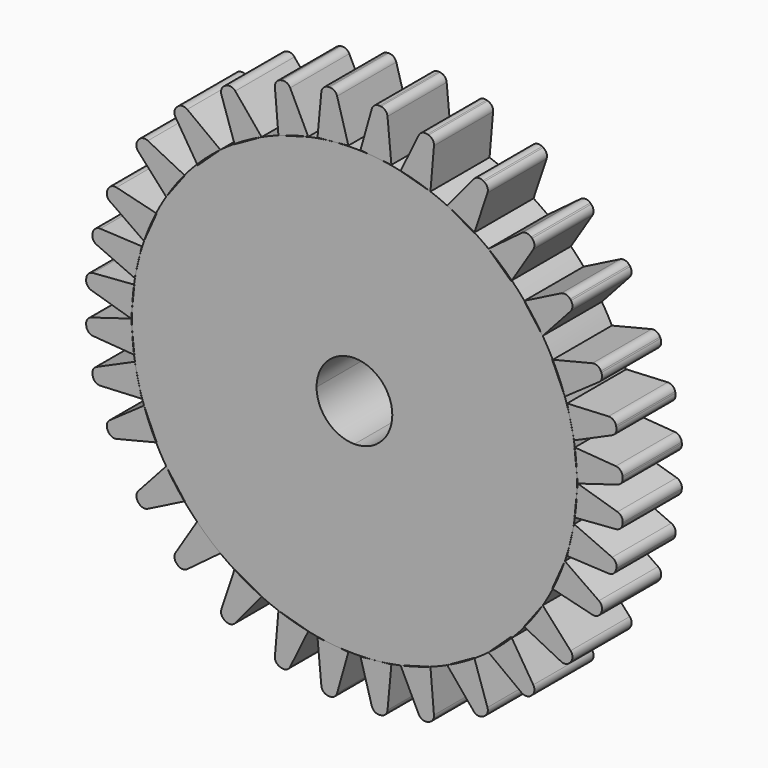
from build123d import *

# Parameters (mm, degrees)
F1_DEPTH = 12.7
F2_DEPTH = 12.7


# Not quite as in the source:
# - a feature names something its author has since deleted; it is built from what else it names


with BuildPart() as f1:
    # F0 (on Front) → F1 (new body)
    with BuildSketch(Plane.XZ):
        with BuildLine():
            Line((6.5054095145, 0), (38.2263594969, 0))
            ThreePointArc((38.2263594969, 0), (38.2190910967, 0.7454100379), (38.1972886603, 1.4905366096))
            Line((38.1972886603, 1.4905366096), (37.8051740161, 5.3060541003))
            Line((37.8051740161, 5.3060541003), (37.8568663972, 5.3020964693))
            ThreePointArc((37.8568663972, 5.3020964693), (37.7123171402, 6.247855336), (37.5441442564, 7.1897004415))
            Line((37.5441442564, 7.1897004415), (36.8769989926, 10.0668518258))
            ThreePointArc((36.8769989926, 10.0668518258), (36.5302837796, 11.2602365592), (36.1449602441, 12.4417205133))
            Line((36.1449602441, 12.4417205133), (33.966945199, 17.3107867958))
            Line((33.966945199, 17.3107867958), (34.0692924567, 17.3360281461))
            ThreePointArc((34.0692924567, 17.3360281461), (33.2407623999, 18.8760768026), (32.3426638377, 20.3766203347))
            Line((32.3426638377, 20.3766203347), (29.136457273, 24.6303906457))
            Line((29.136457273, 24.6303906457), (29.2045556993, 24.6647215023))
            ThreePointArc((29.2045556993, 24.6647215023), (28.1414113561, 25.8711330882), (27.0284704993, 27.0317654409))
            Line((27.0284704993, 27.0317654409), (26.9292951534, 26.873760444))
            Line((26.9292951534, 26.873760444), (23.028254509, 30.5115396965))
            ThreePointArc((23.028254509, 30.5115396965), (21.8357551707, 31.3760156251), (20.6108385483, 32.193910833))
            Line((20.6108385483, 32.193910833), (20.5898791317, 32.1310935588))
            Line((20.5898791317, 32.1310935588), (15.9399155527, 34.7444046223))
            ThreePointArc((15.9399155527, 34.7444046223), (14.4762769158, 35.3792589951), (12.9874228564, 35.9524882022))
            Line((12.9874228564, 35.9524882022), (7.9227071255, 37.3802185059))
            Line((7.9227071255, 37.3802185059), (7.9298244174, 37.3948184257))
            ThreePointArc((7.9298244174, 37.3948184257), (6.2217980358, 37.7166248435), (4.5009090674, 37.960458084))
            Line((4.5009090674, 37.960458084), (2.9038043086, 38.1159085018))
            ThreePointArc((2.9038043086, 38.1159085018), (0, 38.2263594969), (-2.9038043086, 38.1159085018))
            Line((-2.9038043086, 38.1159085018), (-4.5009090674, 37.960458084))
            ThreePointArc((-4.5009090674, 37.960458084), (-6.2217980358, 37.7166248435), (-7.9298244174, 37.3948184257))
            Line((-7.9298244174, 37.3948184257), (-7.9227071255, 37.3802185059))
            Line((-7.9227071255, 37.3802185059), (-12.9874228564, 35.9524882022))
            ThreePointArc((-12.9874228564, 35.9524882022), (-14.4762769158, 35.3792589951), (-15.9399155527, 34.7444046223))
            Line((-15.9399155527, 34.7444046223), (-20.5898791317, 32.1310935588))
            Line((-20.5898791317, 32.1310935588), (-20.6108385483, 32.193910833))
            ThreePointArc((-20.6108385483, 32.193910833), (-21.8357551707, 31.3760156251), (-23.028254509, 30.5115396965))
            Line((-23.028254509, 30.5115396965), (-26.9292951534, 26.873760444))
            Line((-26.9292951534, 26.873760444), (-27.0284704993, 27.0317654409))
            ThreePointArc((-27.0284704993, 27.0317654409), (-28.1414113561, 25.8711330882), (-29.2045556993, 24.6647215023))
            Line((-29.2045556993, 24.6647215023), (-29.136457273, 24.6303906457))
            Line((-29.136457273, 24.6303906457), (-32.3426638377, 20.3766203347))
            ThreePointArc((-32.3426638377, 20.3766203347), (-33.2407623999, 18.8760768026), (-34.0692924567, 17.3360281461))
            Line((-34.0692924567, 17.3360281461), (-33.966945199, 17.3107867958))
            Line((-33.966945199, 17.3107867958), (-36.1449602441, 12.4417205133))
            ThreePointArc((-36.1449602441, 12.4417205133), (-36.5302837796, 11.2602365592), (-36.8769989926, 10.0668518258))
            Line((-36.8769989926, 10.0668518258), (-37.5441442564, 7.1897004415))
            ThreePointArc((-37.5441442564, 7.1897004415), (-37.7123171402, 6.247855336), (-37.8568663972, 5.3020964693))
            Line((-37.8568663972, 5.3020964693), (-37.8051740161, 5.3060541003))
            Line((-37.8051740161, 5.3060541003), (-38.1972886603, 1.4905366096))
            ThreePointArc((-38.1972886603, 1.4905366096), (-38.2190910967, 0.7454100379), (-38.2263594969, 0))
            Line((-38.2263594969, 0), (-6.5054095145, 0))
            ThreePointArc((-6.5054095145, 0), (-4.6000191821, 4.6000191821), (0, 6.5054095145))
            ThreePointArc((0, 6.5054095145), (4.6000191821, 4.6000191821), (6.5054095145, 0))
        make_face()
        with BuildLine():
            Line((0, -38.2263594969), (0, -6.5054095145))
            ThreePointArc((0, -6.5054095145), (-4.6000191821, -4.6000191821), (-6.5054095145, 0))
            Line((-6.5054095145, 0), (-38.2263594969, 0))
            ThreePointArc((-38.2263594969, 0), (-38.2190910967, -0.7454100379), (-38.1972886603, -1.4905366096))
            Line((-38.1972886603, -1.4905366096), (-37.8051740161, -5.3060541003))
            Line((-37.8051740161, -5.3060541003), (-37.8568663972, -5.3020964693))
            ThreePointArc((-37.8568663972, -5.3020964693), (-37.7123171402, -6.247855336), (-37.5441442564, -7.1897004415))
            Line((-37.5441442564, -7.1897004415), (-36.8769989926, -10.0668518258))
            ThreePointArc((-36.8769989926, -10.0668518258), (-36.5302837796, -11.2602365592), (-36.1449602441, -12.4417205133))
            Line((-36.1449602441, -12.4417205133), (-33.966945199, -17.3107867958))
            Line((-33.966945199, -17.3107867958), (-34.0692924567, -17.3360281461))
            ThreePointArc((-34.0692924567, -17.3360281461), (-33.2407623999, -18.8760768026), (-32.3426638377, -20.3766203347))
            Line((-32.3426638377, -20.3766203347), (-29.136457273, -24.6303906457))
            Line((-29.136457273, -24.6303906457), (-29.2045556993, -24.6647215023))
            ThreePointArc((-29.2045556993, -24.6647215023), (-28.1414113561, -25.8711330882), (-27.0284704993, -27.0317654409))
            ThreePointArc((-27.0284704993, -27.0317654409), (-25.0887651521, -28.8410891529), (-23.028254509, -30.5115396965))
            ThreePointArc((-23.028254509, -30.5115396965), (-21.8357551707, -31.3760156251), (-20.6108385483, -32.193910833))
            Line((-20.6108385483, -32.193910833), (-20.5898791317, -32.1310935588))
            Line((-20.5898791317, -32.1310935588), (-15.9399155527, -34.7444046223))
            ThreePointArc((-15.9399155527, -34.7444046223), (-14.4762769158, -35.3792589951), (-12.9874228564, -35.9524882022))
            Line((-12.9874228564, -35.9524882022), (-7.9227071255, -37.3802185059))
            Line((-7.9227071255, -37.3802185059), (-7.9298244174, -37.3948184257))
            ThreePointArc((-7.9298244174, -37.3948184257), (-6.2217980358, -37.7166248435), (-4.5009090674, -37.960458084))
            Line((-4.5009090674, -37.960458084), (-2.9038043086, -38.1159085018))
            ThreePointArc((-2.9038043086, -38.1159085018), (-1.4529520712, -38.1987367679), (0, -38.2263594969))
        make_face()
        with BuildLine():
            ThreePointArc((38.1972886603, -1.4905366096), (38.2190910967, -0.7454100379), (38.2263594969, 0))
            Line((38.2263594969, 0), (6.5054095145, 0))
            ThreePointArc((6.5054095145, 0), (4.6000191821, -4.6000191821), (0, -6.5054095145))
            Line((0, -6.5054095145), (0, -38.2263594969))
            ThreePointArc((0, -38.2263594969), (1.4529520712, -38.1987367679), (2.9038043086, -38.1159085018))
            Line((2.9038043086, -38.1159085018), (4.5009090674, -37.960458084))
            ThreePointArc((4.5009090674, -37.960458084), (6.2217980358, -37.7166248435), (7.9298244174, -37.3948184257))
            Line((7.9298244174, -37.3948184257), (7.9227071255, -37.3802185059))
            Line((7.9227071255, -37.3802185059), (12.9874228564, -35.9524882022))
            ThreePointArc((12.9874228564, -35.9524882022), (14.4762769158, -35.3792589951), (15.9399155527, -34.7444046223))
            Line((15.9399155527, -34.7444046223), (20.5898791317, -32.1310935588))
            Line((20.5898791317, -32.1310935588), (20.6108385483, -32.193910833))
            ThreePointArc((20.6108385483, -32.193910833), (21.8357551707, -31.3760156251), (23.028254509, -30.5115396965))
            Line((23.028254509, -30.5115396965), (26.9292951534, -26.873760444))
            Line((26.9292951534, -26.873760444), (27.0284704993, -27.0317654409))
            ThreePointArc((27.0284704993, -27.0317654409), (28.1414113561, -25.8711330882), (29.2045556993, -24.6647215023))
            Line((29.2045556993, -24.6647215023), (29.136457273, -24.6303906457))
            Line((29.136457273, -24.6303906457), (32.3426638377, -20.3766203347))
            ThreePointArc((32.3426638377, -20.3766203347), (33.2407623999, -18.8760768026), (34.0692924567, -17.3360281461))
            Line((34.0692924567, -17.3360281461), (33.966945199, -17.3107867958))
            Line((33.966945199, -17.3107867958), (36.1449602441, -12.4417205133))
            ThreePointArc((36.1449602441, -12.4417205133), (36.5302837796, -11.2602365592), (36.8769989926, -10.0668518258))
            Line((36.8769989926, -10.0668518258), (37.5441442564, -7.1897004415))
            ThreePointArc((37.5441442564, -7.1897004415), (37.7123171402, -6.247855336), (37.8568663972, -5.3020964693))
            Line((37.8568663972, -5.3020964693), (37.8051740161, -5.3060541003))
            Line((37.8051740161, -5.3060541003), (38.1972886603, -1.4905366096))
        make_face()
    extrude(amount=F1_DEPTH)


with BuildPart() as f2:
    # F0 (on Front) → F2 (new body)
    with BuildSketch(Plane.XZ):
        with BuildLine():
            ThreePointArc((7.9298244174, 37.3948184257), (10.4834578025, 36.760735478), (12.9874228564, 35.9524882022))
            Line((12.9874228564, 35.9524882022), (13.0566200219, 35.9329816997))
            Line((13.0566200219, 35.9329816997), (13.6614098518, 43.048311445))
            ThreePointArc((13.6614098518, 43.048311445), (13.4401043597, 43.8788438049), (12.7405530088, 44.3782314591))
            Line((12.7405530088, 44.3782314591), (12.5253001319, 44.43891069))
            ThreePointArc((12.5253001319, 44.43891069), (11.6614494202, 44.3755406091), (11.0391416998, 43.7730566505))
            Line((11.0391416998, 43.7730566505), (7.9298244174, 37.3948184257))
        make_face()
    extrude(amount=F2_DEPTH)


with BuildPart() as f2b:
    # F0 (on Front) → F2, piece 2 (new body)
    with BuildSketch(Plane.XZ):
        with BuildLine():
            ThreePointArc((2.9038043086, 38.1159085018), (3.703172458, 38.046564551), (4.5009090674, 37.960458084))
            Line((4.5009090674, 37.960458084), (6.3482185459, 37.7806545811))
            Line((6.3482185459, 37.7806545811), (5.6854478482, 44.8908179494))
            ThreePointArc((5.6854478482, 44.8908179494), (5.320785814, 45.6691377567), (4.5439606825, 46.0369730958))
            Line((4.5439606825, 46.0369730958), (4.3213705089, 46.0586383843))
            ThreePointArc((4.3213705089, 46.0586383843), (3.4823333385, 45.8435327225), (2.976352358, 45.1405127607))
            Line((2.976352358, 45.1405127607), (1.0393066332, 38.2973849773))
            Line((1.0393066332, 38.2973849773), (2.9038043086, 38.1159085018))
        make_face()
    extrude(amount=F2_DEPTH)


with BuildPart() as f2c:
    # F0 (on Front) → F2, piece 3 (new body)
    with BuildSketch(Plane.XZ):
        with BuildLine():
            ThreePointArc((-4.5009090674, 37.960458084), (-3.703172458, 38.046564551), (-2.9038043086, 38.1159085018))
            Line((-2.9038043086, 38.1159085018), (-1.0393066332, 38.2973849773))
            Line((-1.0393066332, 38.2973849773), (-2.976352358, 45.1405127607))
            ThreePointArc((-2.976352358, 45.1405127607), (-3.4823333385, 45.8435327225), (-4.3213705089, 46.0586383843))
            Line((-4.3213705089, 46.0586383843), (-4.5439606825, 46.0369730958))
            ThreePointArc((-4.5439606825, 46.0369730958), (-5.320785814, 45.6691377567), (-5.6854478482, 44.8908179494))
            Line((-5.6854478482, 44.8908179494), (-6.3482185459, 37.7806545811))
            Line((-6.3482185459, 37.7806545811), (-4.5009090674, 37.960458084))
        make_face()
    extrude(amount=F2_DEPTH)


with BuildPart() as f2d:
    # F0 (on Front) → F2, piece 4 (new body)
    with BuildSketch(Plane.XZ):
        with BuildLine():
            Line((-13.0566200219, 35.9329816997), (-12.9874228564, 35.9524882022))
            ThreePointArc((-12.9874228564, 35.9524882022), (-10.4834578025, 36.760735478), (-7.9298244174, 37.3948184257))
            Line((-7.9298244174, 37.3948184257), (-11.0391416998, 43.7730566505))
            ThreePointArc((-11.0391416998, 43.7730566505), (-11.6614494202, 44.3755406091), (-12.5253001319, 44.43891069))
            Line((-12.5253001319, 44.43891069), (-12.7405530088, 44.3782314591))
            ThreePointArc((-12.7405530088, 44.3782314591), (-13.4401043597, 43.8788438049), (-13.6614098518, 43.048311445))
            Line((-13.6614098518, 43.048311445), (-13.0566200219, 35.9329816997))
        make_face()
    extrude(amount=F2_DEPTH)


with BuildPart() as f2e:
    # F0 (on Front) → F2, piece 5 (new body)
    with BuildSketch(Plane.XZ):
        with BuildLine():
            Line((-22.8500298253, 38.9049703635), (-20.6108385483, 32.193910833))
            ThreePointArc((-20.6108385483, 32.193910833), (-18.3198160739, 33.5505424606), (-15.9399155527, 34.7444046223))
            Line((-15.9399155527, 34.7444046223), (-20.4715505207, 40.2257209347))
            ThreePointArc((-20.4715505207, 40.2257209347), (-21.2180271407, 40.6650687184), (-22.0725739249, 40.5236345902))
            Line((-22.0725739249, 40.5236345902), (-22.2675359467, 40.4140646118))
            ThreePointArc((-22.2675359467, 40.4140646118), (-22.8301217888, 39.7642513371), (-22.8500298253, 38.9049703635))
        make_face()
    extrude(amount=F2_DEPTH)


with BuildPart() as f2f:
    # F0 (on Front) → F2, piece 6 (new body)
    with BuildSketch(Plane.XZ):
        with BuildLine():
            Line((-30.7256257514, 32.9220297925), (-27.0284704993, 27.0317654409))
            ThreePointArc((-27.0284704993, 27.0317654409), (-25.0887651521, 28.8410891529), (-23.028254509, 30.5115396965))
            Line((-23.028254509, 30.5115396965), (-28.7264515234, 34.76725289))
            ThreePointArc((-28.7264515234, 34.76725289), (-29.5555860309, 35.0178317951), (-30.3525382252, 34.6785369099))
            Line((-30.3525382252, 34.6785369099), (-30.5160996721, 34.5260133932))
            ThreePointArc((-30.5160996721, 34.5260133932), (-30.9092629563, 33.7616949035), (-30.7256257514, 32.9220297925))
        make_face()
    extrude(amount=F2_DEPTH)


with BuildPart() as f2g:
    # F0 (on Front) → F2, piece 7 (new body)
    with BuildSketch(Plane.XZ):
        with BuildLine():
            Line((-37.1311925638, 25.6733367197), (-32.3426638377, 20.3766203347))
            ThreePointArc((-32.3426638377, 20.3766203347), (-30.8482092039, 22.5752641024), (-29.2045556993, 24.6647215023))
            Line((-29.2045556993, 24.6647215023), (-35.4870827117, 27.8319684657))
            ThreePointArc((-35.4870827117, 27.8319684657), (-36.3470628398, 27.9347792591), (-37.0729729559, 27.4623489643))
            Line((-37.0729729559, 27.4623489643), (-37.2032913071, 27.2894517032))
            ThreePointArc((-37.2032913071, 27.2894517032), (-37.4578494531, 26.4684295171), (-37.1311925638, 25.6733367197))
        make_face()
    extrude(amount=F2_DEPTH)


with BuildPart() as f2h:
    # F0 (on Front) → F2, piece 8 (new body)
    with BuildSketch(Plane.XZ):
        with BuildLine():
            Line((-41.9956275532, 16.5360312198), (-36.1449602441, 12.4417205133))
            ThreePointArc((-36.1449602441, 12.4417205133), (-35.1923128309, 14.9250017755), (-34.0692924567, 17.3360281461))
            Line((-34.0692924567, 17.3360281461), (-40.8720479211, 19.0137549098))
            ThreePointArc((-40.8720479211, 19.0137549098), (-41.7333404119, 18.9219449729), (-42.3354508659, 18.299275863))
            Line((-42.3354508659, 18.299275863), (-42.4267699073, 18.0951273809))
            ThreePointArc((-42.4267699073, 18.0951273809), (-42.4915281014, 17.2380588317), (-41.9956275532, 16.5360312198))
        make_face()
    extrude(amount=F2_DEPTH)


with BuildPart() as f2i:
    # F0 (on Front) → F2, piece 9 (new body)
    with BuildSketch(Plane.XZ):
        with BuildLine():
            Line((-37.7432952731, 6.3308355817), (-37.5441442564, 7.1897004415))
            ThreePointArc((-37.5441442564, 7.1897004415), (-37.2383691996, 8.6347217523), (-36.8769989926, 10.0668518258))
            Line((-36.8769989926, 10.0668518258), (-36.5384301896, 11.5269741605))
            Line((-36.5384301896, 11.5269741605), (-43.6418837203, 11.8755310958))
            ThreePointArc((-43.6418837203, 11.8755310958), (-44.4696339916, 11.6204167929), (-44.9413018823, 10.89392989))
            Line((-44.9413018823, 10.89392989), (-44.9918190377, 10.6760680367))
            ThreePointArc((-44.9918190377, 10.6760680367), (-44.8911820225, 9.8224684158), (-44.2699736332, 9.2284479964))
            Line((-44.2699736332, 9.2284479964), (-37.7432952731, 6.3308355817))
        make_face()
    extrude(amount=F2_DEPTH)


with BuildPart() as f2j:
    # F0 (on Front) → F2, piece 10 (new body)
    with BuildSketch(Plane.XZ):
        with BuildLine():
            Line((-38.3504687251, 4.1e-08), (-38.1972886603, 1.4905366096))
            ThreePointArc((-38.1972886603, 1.4905366096), (-38.0748029872, 3.4005790486), (-37.8568663972, 5.3020964693))
            Line((-37.8568663972, 5.3020964693), (-44.8964212907, 4.7631396591))
            ThreePointArc((-44.8964212907, 4.7631396591), (-45.6857494873, 4.406467797), (-46.062818488, 3.6266775765))
            Line((-46.062818488, 3.6266775765), (-46.0856814109, 3.404207226))
            ThreePointArc((-46.0856814109, 3.404207226), (-45.8790389527, 2.5699057121), (-45.1883921618, 2.0582738798))
            Line((-45.1883921618, 2.0582738798), (-38.3504687251, 4.1e-08))
        make_face()
    extrude(amount=F2_DEPTH)


with BuildPart() as f2k:
    # F0 (on Front) → F2, piece 11 (new body)
    with BuildSketch(Plane.XZ):
        with BuildLine():
            ThreePointArc((-37.8568663972, -5.3020964693), (-38.0748029872, -3.4005790486), (-38.1972886603, -1.4905366096))
            Line((-38.1972886603, -1.4905366096), (-38.3504687251, -4.1e-08))
            Line((-38.3504687251, -4.1e-08), (-45.1883921618, -2.0582738798))
            ThreePointArc((-45.1883921618, -2.0582738798), (-45.8790389527, -2.5699057121), (-46.0856814109, -3.404207226))
            Line((-46.0856814109, -3.404207226), (-46.062818488, -3.6266775765))
            ThreePointArc((-46.062818488, -3.6266775765), (-45.6857494873, -4.406467797), (-44.8964212907, -4.7631396591))
            Line((-44.8964212907, -4.7631396591), (-37.8568663972, -5.3020964693))
        make_face()
    extrude(amount=F2_DEPTH)


with BuildPart() as f2l:
    # F0 (on Front) → F2, piece 12 (new body)
    with BuildSketch(Plane.XZ):
        with BuildLine():
            ThreePointArc((-36.8769989926, -10.0668518258), (-37.2383691996, -8.6347217523), (-37.5441442564, -7.1897004415))
            Line((-37.5441442564, -7.1897004415), (-37.7432952731, -6.3308355817))
            Line((-37.7432952731, -6.3308355817), (-44.2699736332, -9.2284479964))
            ThreePointArc((-44.2699736332, -9.2284479964), (-44.8911820225, -9.8224684158), (-44.9918190377, -10.6760680367))
            Line((-44.9918190377, -10.6760680367), (-44.9413018823, -10.89392989))
            ThreePointArc((-44.9413018823, -10.89392989), (-44.4696339916, -11.6204167929), (-43.6418837203, -11.8755310958))
            Line((-43.6418837203, -11.8755310958), (-36.5384301896, -11.5269741605))
            Line((-36.5384301896, -11.5269741605), (-36.8769989926, -10.0668518258))
        make_face()
    extrude(amount=F2_DEPTH)


with BuildPart() as f2m:
    # F0 (on Front) → F2, piece 13 (new body)
    with BuildSketch(Plane.XZ):
        with BuildLine():
            ThreePointArc((-34.0692924567, -17.3360281461), (-35.1923128309, -14.9250017755), (-36.1449602441, -12.4417205133))
            Line((-36.1449602441, -12.4417205133), (-41.9956275532, -16.5360312198))
            ThreePointArc((-41.9956275532, -16.5360312198), (-42.4915281014, -17.2380588317), (-42.4267699073, -18.0951273809))
            Line((-42.4267699073, -18.0951273809), (-42.3354508659, -18.299275863))
            ThreePointArc((-42.3354508659, -18.299275863), (-41.7333404119, -18.9219449729), (-40.8720479211, -19.0137549098))
            Line((-40.8720479211, -19.0137549098), (-34.0692924567, -17.3360281461))
        make_face()
    extrude(amount=F2_DEPTH)


with BuildPart() as f2n:
    # F0 (on Front) → F2, piece 14 (new body)
    with BuildSketch(Plane.XZ):
        with BuildLine():
            ThreePointArc((-29.2045556993, -24.6647215023), (-30.8482092039, -22.5752641024), (-32.3426638377, -20.3766203347))
            Line((-32.3426638377, -20.3766203347), (-37.1311925638, -25.6733367197))
            ThreePointArc((-37.1311925638, -25.6733367197), (-37.4578494531, -26.4684295171), (-37.2032913071, -27.2894517032))
            Line((-37.2032913071, -27.2894517032), (-37.0729729559, -27.4623489643))
            ThreePointArc((-37.0729729559, -27.4623489643), (-36.3470628398, -27.9347792591), (-35.4870827117, -27.8319684657))
            Line((-35.4870827117, -27.8319684657), (-29.2045556993, -24.6647215023))
        make_face()
    extrude(amount=F2_DEPTH)


with BuildPart() as f2o:
    # F0 (on Front) → F2, piece 15 (new body)
    with BuildSketch(Plane.XZ):
        with BuildLine():
            Line((-28.7264515234, -34.76725289), (-23.028254509, -30.5115396965))
            ThreePointArc((-23.028254509, -30.5115396965), (-25.0887651521, -28.8410891529), (-27.0284704993, -27.0317654409))
            Line((-27.0284704993, -27.0317654409), (-30.7256257514, -32.9220297925))
            ThreePointArc((-30.7256257514, -32.9220297925), (-30.9092629563, -33.7616949035), (-30.5160996721, -34.5260133932))
            Line((-30.5160996721, -34.5260133932), (-30.3525382252, -34.6785369099))
            ThreePointArc((-30.3525382252, -34.6785369099), (-29.5555860309, -35.0178317951), (-28.7264515234, -34.76725289))
        make_face()
    extrude(amount=F2_DEPTH)


with BuildPart() as f2p:
    # F0 (on Front) → F2, piece 16 (new body)
    with BuildSketch(Plane.XZ):
        with BuildLine():
            Line((-20.4715505207, -40.2257209347), (-15.9399155527, -34.7444046223))
            ThreePointArc((-15.9399155527, -34.7444046223), (-18.3198160739, -33.5505424606), (-20.6108385483, -32.193910833))
            Line((-20.6108385483, -32.193910833), (-22.8500298253, -38.9049703635))
            ThreePointArc((-22.8500298253, -38.9049703635), (-22.8301217888, -39.7642513371), (-22.2675359467, -40.4140646118))
            Line((-22.2675359467, -40.4140646118), (-22.0725739249, -40.5236345902))
            ThreePointArc((-22.0725739249, -40.5236345902), (-21.2180271407, -40.6650687184), (-20.4715505207, -40.2257209347))
        make_face()
    extrude(amount=F2_DEPTH)


with BuildPart() as f2q:
    # F0 (on Front) → F2, piece 17 (new body)
    with BuildSketch(Plane.XZ):
        with BuildLine():
            Line((-11.0391416998, -43.7730566505), (-7.9298244174, -37.3948184257))
            ThreePointArc((-7.9298244174, -37.3948184257), (-10.4834578025, -36.760735478), (-12.9874228564, -35.9524882022))
            Line((-12.9874228564, -35.9524882022), (-13.0566200219, -35.9329816997))
            Line((-13.0566200219, -35.9329816997), (-13.6614098518, -43.048311445))
            ThreePointArc((-13.6614098518, -43.048311445), (-13.4401043597, -43.8788438049), (-12.7405530088, -44.3782314591))
            Line((-12.7405530088, -44.3782314591), (-12.5253001319, -44.43891069))
            ThreePointArc((-12.5253001319, -44.43891069), (-11.6614494202, -44.3755406091), (-11.0391416998, -43.7730566505))
        make_face()
    extrude(amount=F2_DEPTH)


with BuildPart() as f2r:
    # F0 (on Front) → F2, piece 18 (new body)
    with BuildSketch(Plane.XZ):
        with BuildLine():
            Line((-1.0393066332, -38.2973849773), (-2.9038043086, -38.1159085018))
            ThreePointArc((-2.9038043086, -38.1159085018), (-3.703172458, -38.046564551), (-4.5009090674, -37.960458084))
            Line((-4.5009090674, -37.960458084), (-6.3482185459, -37.7806545811))
            Line((-6.3482185459, -37.7806545811), (-5.6854478482, -44.8908179494))
            ThreePointArc((-5.6854478482, -44.8908179494), (-5.320785814, -45.6691377567), (-4.5439606825, -46.0369730958))
            Line((-4.5439606825, -46.0369730958), (-4.3213705089, -46.0586383843))
            ThreePointArc((-4.3213705089, -46.0586383843), (-3.4823333385, -45.8435327225), (-2.976352358, -45.1405127607))
            Line((-2.976352358, -45.1405127607), (-1.0393066332, -38.2973849773))
        make_face()
    extrude(amount=F2_DEPTH)


with BuildPart() as f2s:
    # F0 (on Front) → F2, piece 19 (new body)
    with BuildSketch(Plane.XZ):
        with BuildLine():
            ThreePointArc((4.5009090674, -37.960458084), (3.703172458, -38.046564551), (2.9038043086, -38.1159085018))
            Line((2.9038043086, -38.1159085018), (1.0393066332, -38.2973849773))
            Line((1.0393066332, -38.2973849773), (2.976352358, -45.1405127607))
            ThreePointArc((2.976352358, -45.1405127607), (3.4823333385, -45.8435327225), (4.3213705089, -46.0586383843))
            Line((4.3213705089, -46.0586383843), (4.5439606825, -46.0369730958))
            ThreePointArc((4.5439606825, -46.0369730958), (5.320785814, -45.6691377567), (5.6854478482, -44.8908179494))
            Line((5.6854478482, -44.8908179494), (6.3482185459, -37.7806545811))
            Line((6.3482185459, -37.7806545811), (4.5009090674, -37.960458084))
        make_face()
    extrude(amount=F2_DEPTH)


with BuildPart() as f2t:
    # F0 (on Front) → F2, piece 20 (new body)
    with BuildSketch(Plane.XZ):
        with BuildLine():
            ThreePointArc((12.9874228564, -35.9524882022), (10.4834578025, -36.760735478), (7.9298244174, -37.3948184257))
            Line((7.9298244174, -37.3948184257), (11.0391416998, -43.7730566505))
            ThreePointArc((11.0391416998, -43.7730566505), (11.6614494202, -44.3755406091), (12.5253001319, -44.43891069))
            Line((12.5253001319, -44.43891069), (12.7405530088, -44.3782314591))
            ThreePointArc((12.7405530088, -44.3782314591), (13.4401043597, -43.8788438049), (13.6614098518, -43.048311445))
            Line((13.6614098518, -43.048311445), (13.0566200219, -35.9329816997))
            Line((13.0566200219, -35.9329816997), (12.9874228564, -35.9524882022))
        make_face()
    extrude(amount=F2_DEPTH)


with BuildPart() as f2u:
    # F0 (on Front) → F2, piece 21 (new body)
    with BuildSketch(Plane.XZ):
        with BuildLine():
            ThreePointArc((20.6108385483, -32.193910833), (18.3198160739, -33.5505424606), (15.9399155527, -34.7444046223))
            Line((15.9399155527, -34.7444046223), (20.4715505207, -40.2257209347))
            ThreePointArc((20.4715505207, -40.2257209347), (21.2180271407, -40.6650687184), (22.0725739249, -40.5236345902))
            Line((22.0725739249, -40.5236345902), (22.2675359467, -40.4140646118))
            ThreePointArc((22.2675359467, -40.4140646118), (22.8301217888, -39.7642513371), (22.8500298253, -38.9049703635))
            Line((22.8500298253, -38.9049703635), (20.6108385483, -32.193910833))
        make_face()
    extrude(amount=F2_DEPTH)


with BuildPart() as f2v:
    # F0 (on Front) → F2, piece 22 (new body)
    with BuildSketch(Plane.XZ):
        with BuildLine():
            Line((30.7256257514, -32.9220297925), (27.0284704993, -27.0317654409))
            ThreePointArc((27.0284704993, -27.0317654409), (25.0887651521, -28.8410891529), (23.028254509, -30.5115396965))
            Line((23.028254509, -30.5115396965), (28.7264515234, -34.76725289))
            ThreePointArc((28.7264515234, -34.76725289), (29.5555860309, -35.0178317951), (30.3525382252, -34.6785369099))
            Line((30.3525382252, -34.6785369099), (30.5160996721, -34.5260133932))
            ThreePointArc((30.5160996721, -34.5260133932), (30.9092629563, -33.7616949035), (30.7256257514, -32.9220297925))
        make_face()
    extrude(amount=F2_DEPTH)


with BuildPart() as f2w:
    # F0 (on Front) → F2, piece 23 (new body)
    with BuildSketch(Plane.XZ):
        with BuildLine():
            Line((37.1311925638, -25.6733367197), (32.3426638377, -20.3766203347))
            ThreePointArc((32.3426638377, -20.3766203347), (30.8482092039, -22.5752641024), (29.2045556993, -24.6647215023))
            Line((29.2045556993, -24.6647215023), (35.4870827117, -27.8319684657))
            ThreePointArc((35.4870827117, -27.8319684657), (36.3470628398, -27.9347792591), (37.0729729559, -27.4623489643))
            Line((37.0729729559, -27.4623489643), (37.2032913071, -27.2894517032))
            ThreePointArc((37.2032913071, -27.2894517032), (37.4578494531, -26.4684295171), (37.1311925638, -25.6733367197))
        make_face()
    extrude(amount=F2_DEPTH)


with BuildPart() as f2x:
    # F0 (on Front) → F2, piece 24 (new body)
    with BuildSketch(Plane.XZ):
        with BuildLine():
            Line((41.9956275532, -16.5360312198), (36.1449602441, -12.4417205133))
            ThreePointArc((36.1449602441, -12.4417205133), (35.1923128309, -14.9250017755), (34.0692924567, -17.3360281461))
            Line((34.0692924567, -17.3360281461), (40.8720479211, -19.0137549098))
            ThreePointArc((40.8720479211, -19.0137549098), (41.7333404119, -18.9219449729), (42.3354508659, -18.299275863))
            Line((42.3354508659, -18.299275863), (42.4267699073, -18.0951273809))
            ThreePointArc((42.4267699073, -18.0951273809), (42.4915281014, -17.2380588317), (41.9956275532, -16.5360312198))
        make_face()
    extrude(amount=F2_DEPTH)


with BuildPart() as f2y:
    # F0 (on Front) → F2, piece 25 (new body)
    with BuildSketch(Plane.XZ):
        with BuildLine():
            Line((37.7432952731, -6.3308355817), (37.5441442564, -7.1897004415))
            ThreePointArc((37.5441442564, -7.1897004415), (37.2383691996, -8.6347217523), (36.8769989926, -10.0668518258))
            Line((36.8769989926, -10.0668518258), (36.5384301896, -11.5269741605))
            Line((36.5384301896, -11.5269741605), (43.6418837203, -11.8755310958))
            ThreePointArc((43.6418837203, -11.8755310958), (44.4696339916, -11.6204167929), (44.9413018823, -10.89392989))
            Line((44.9413018823, -10.89392989), (44.9918190377, -10.6760680367))
            ThreePointArc((44.9918190377, -10.6760680367), (44.8911820225, -9.8224684158), (44.2699736332, -9.2284479964))
            Line((44.2699736332, -9.2284479964), (37.7432952731, -6.3308355817))
        make_face()
    extrude(amount=F2_DEPTH)


with BuildPart() as f2z:
    # F0 (on Front) → F2, piece 26 (new body)
    with BuildSketch(Plane.XZ):
        with BuildLine():
            Line((38.3504687251, -4.1e-08), (38.1972886603, -1.4905366096))
            ThreePointArc((38.1972886603, -1.4905366096), (38.0748029872, -3.4005790486), (37.8568663972, -5.3020964693))
            Line((37.8568663972, -5.3020964693), (44.8964212907, -4.7631396591))
            ThreePointArc((44.8964212907, -4.7631396591), (45.6857494873, -4.406467797), (46.062818488, -3.6266775765))
            Line((46.062818488, -3.6266775765), (46.0856814109, -3.404207226))
            ThreePointArc((46.0856814109, -3.404207226), (45.8790389527, -2.5699057121), (45.1883921618, -2.0582738798))
            Line((45.1883921618, -2.0582738798), (38.3504687251, -4.1e-08))
        make_face()
    extrude(amount=F2_DEPTH)


with BuildPart() as f2ba:
    # F0 (on Front) → F2, piece 27 (new body)
    with BuildSketch(Plane.XZ):
        with BuildLine():
            ThreePointArc((37.8568663972, 5.3020964693), (38.0748029872, 3.4005790486), (38.1972886603, 1.4905366096))
            Line((38.1972886603, 1.4905366096), (38.3504687251, 4.1e-08))
            Line((38.3504687251, 4.1e-08), (45.1883921618, 2.0582738798))
            ThreePointArc((45.1883921618, 2.0582738798), (45.8790389527, 2.5699057121), (46.0856814109, 3.404207226))
            Line((46.0856814109, 3.404207226), (46.062818488, 3.6266775765))
            ThreePointArc((46.062818488, 3.6266775765), (45.6857494873, 4.406467797), (44.8964212907, 4.7631396591))
            Line((44.8964212907, 4.7631396591), (37.8568663972, 5.3020964693))
        make_face()
    extrude(amount=F2_DEPTH)


with BuildPart() as f2bb:
    # F0 (on Front) → F2, piece 28 (new body)
    with BuildSketch(Plane.XZ):
        with BuildLine():
            ThreePointArc((36.8769989926, 10.0668518258), (37.2383691996, 8.6347217523), (37.5441442564, 7.1897004415))
            Line((37.5441442564, 7.1897004415), (37.7432952731, 6.3308355817))
            Line((37.7432952731, 6.3308355817), (44.2699736332, 9.2284479964))
            ThreePointArc((44.2699736332, 9.2284479964), (44.8911820225, 9.8224684158), (44.9918190377, 10.6760680367))
            Line((44.9918190377, 10.6760680367), (44.9413018823, 10.89392989))
            ThreePointArc((44.9413018823, 10.89392989), (44.4696339916, 11.6204167929), (43.6418837203, 11.8755310958))
            Line((43.6418837203, 11.8755310958), (36.5384301896, 11.5269741605))
            Line((36.5384301896, 11.5269741605), (36.8769989926, 10.0668518258))
        make_face()
    extrude(amount=F2_DEPTH)


with BuildPart() as f2bc:
    # F0 (on Front) → F2, piece 29 (new body)
    with BuildSketch(Plane.XZ):
        with BuildLine():
            ThreePointArc((34.0692924567, 17.3360281461), (35.1923128309, 14.9250017755), (36.1449602441, 12.4417205133))
            Line((36.1449602441, 12.4417205133), (41.9956275532, 16.5360312198))
            ThreePointArc((41.9956275532, 16.5360312198), (42.4915281014, 17.2380588317), (42.4267699073, 18.0951273809))
            Line((42.4267699073, 18.0951273809), (42.3354508659, 18.299275863))
            ThreePointArc((42.3354508659, 18.299275863), (41.7333404119, 18.9219449729), (40.8720479211, 19.0137549098))
            Line((40.8720479211, 19.0137549098), (34.0692924567, 17.3360281461))
        make_face()
    extrude(amount=F2_DEPTH)


with BuildPart() as f2bd:
    # F0 (on Front) → F2, piece 30 (new body)
    with BuildSketch(Plane.XZ):
        with BuildLine():
            ThreePointArc((29.2045556993, 24.6647215023), (30.8482092039, 22.5752641024), (32.3426638377, 20.3766203347))
            Line((32.3426638377, 20.3766203347), (37.1311925638, 25.6733367197))
            ThreePointArc((37.1311925638, 25.6733367197), (37.4578494531, 26.4684295171), (37.2032913071, 27.2894517032))
            Line((37.2032913071, 27.2894517032), (37.0729729559, 27.4623489643))
            ThreePointArc((37.0729729559, 27.4623489643), (36.3470628398, 27.9347792591), (35.4870827117, 27.8319684657))
            Line((35.4870827117, 27.8319684657), (29.2045556993, 24.6647215023))
        make_face()
    extrude(amount=F2_DEPTH)


with BuildPart() as f2be:
    # F0 (on Front) → F2, piece 31 (new body)
    with BuildSketch(Plane.XZ):
        with BuildLine():
            ThreePointArc((15.9399155527, 34.7444046223), (18.3198160739, 33.5505424606), (20.6108385483, 32.193910833))
            Line((20.6108385483, 32.193910833), (22.8500298253, 38.9049703635))
            ThreePointArc((22.8500298253, 38.9049703635), (22.8301217888, 39.7642513371), (22.2675359467, 40.4140646118))
            Line((22.2675359467, 40.4140646118), (22.0725739249, 40.5236345902))
            ThreePointArc((22.0725739249, 40.5236345902), (21.2180271407, 40.6650687184), (20.4715505207, 40.2257209347))
            Line((20.4715505207, 40.2257209347), (15.9399155527, 34.7444046223))
        make_face()
    extrude(amount=F2_DEPTH)


with BuildPart() as f2bf:
    # F0 (on Front) → F2, piece 32 (new body)
    with BuildSketch(Plane.XZ):
        with BuildLine():
            ThreePointArc((23.028254509, 30.5115396965), (25.0887651521, 28.8410891529), (27.0284704993, 27.0317654409))
            Line((27.0284704993, 27.0317654409), (30.7256257514, 32.9220297925))
            ThreePointArc((30.7256257514, 32.9220297925), (30.9092629563, 33.7616949035), (30.5160996721, 34.5260133932))
            Line((30.5160996721, 34.5260133932), (30.3525382252, 34.6785369099))
            ThreePointArc((30.3525382252, 34.6785369099), (29.5555860309, 35.0178317951), (28.7264515234, 34.76725289))
            Line((28.7264515234, 34.76725289), (23.028254509, 30.5115396965))
        make_face()
    extrude(amount=F2_DEPTH)


solid = Compound([f1.part, f2.part, f2b.part, f2c.part, f2d.part, f2e.part, f2f.part, f2g.part, f2h.part, f2i.part, f2j.part, f2k.part, f2l.part, f2m.part, f2n.part, f2o.part, f2p.part, f2q.part, f2r.part, f2s.part, f2t.part, f2u.part, f2v.part, f2w.part, f2x.part, f2y.part, f2z.part, f2ba.part, f2bb.part, f2bc.part, f2bd.part, f2be.part, f2bf.part])
